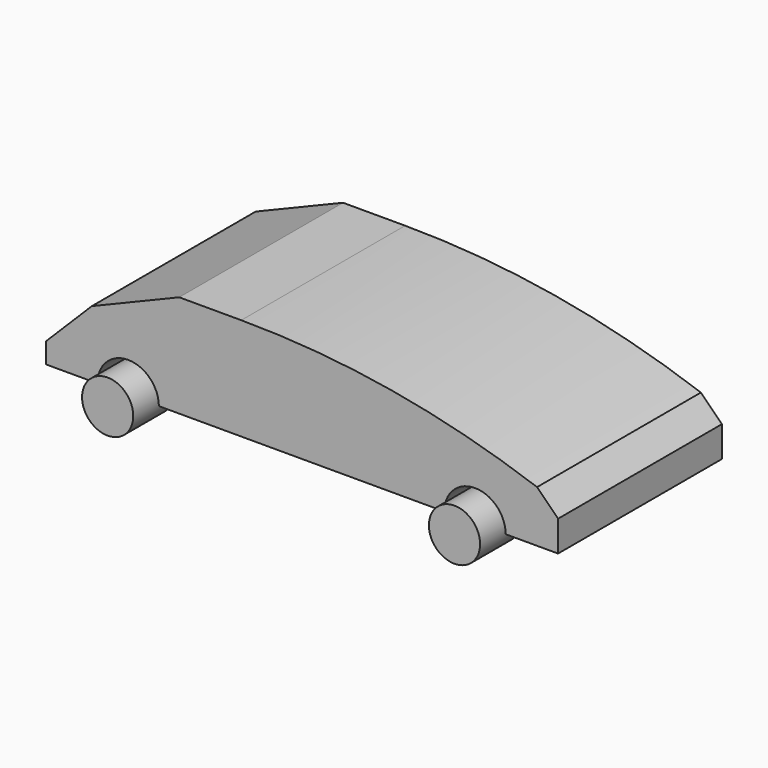
from build123d import *

# Parameters (mm, degrees)
F0_W        = 127
F0_H        = 50.8
F1_DEPTH    = 25.4
F2_SIZE     = 17.78
F3_SIZE     = 17.78
F4_T1_DEPTH = 265.915946003
F5_SIZE     = 20.32
F6_SIZE     = 12.7
F9_DEPTH    = 64.008
F10_DEPTH   = 80.264
F11_DEPTH   = 6.35
F12_R       = 2.54
F13_DEPTH   = 5.08
F15_DEPTH   = 108.712
F16_DEPTH   = 6.35
F17_R       = 2.54
F18_DEPTH   = 5.08
F19_R       = 6.35
F19_R_2     = 2.54
F20_DEPTH   = 6.35
F21_R       = 2.54
F22_DEPTH   = 5.08
F23_DEPTH   = 48.26


# Not quite as in the source:
# - a fillet or chamfer that OpenCascade refuses, or shapes differently, is made with other operations: its cross-section is extruded or revolved along the edge and cut away or added


with BuildPart() as f1:
    # F0 (on Top) → F1 (new body)
    with BuildSketch(Plane.XY):
        with Locations((3.6809762716, -11.9118855059)):
            Rectangle(F0_W, F0_H)
    extrude(amount=F1_DEPTH)

    # F2
    f2_edges = [f1.edges().sort_by_distance(p)[0] for p in [
        (67.180976, -11.911886, 25.4),
    ]]
    chamfer(f2_edges, length=F2_SIZE)

    # F3
    f3_edges = [f1.edges().sort_by_distance(p)[0] for p in [
        (49.400976, -11.911886, 25.4),
    ]]
    chamfer(f3_edges, length=F3_SIZE)

    # F4: fillet of radius 220.4055499979 on 1 edges, made by hand

    # F4_s2 → F4_t1 (cut)
    with BuildSketch(Plane.XZ.offset(-121.0460874956)):
        with BuildLine():
            ThreePointArc((61.9733348411, 12.8276414305), (25.8202104559, 22.2341739644), (-11.402212929, 25.4))
            Line((-11.402212929, 25.4), (31.6209762716, 25.4))
            Line((31.6209762716, 25.4), (61.9733348411, 12.8276414305))
        make_face()
    extrude(amount=F4_T1_DEPTH, mode=Mode.SUBTRACT)

    # F5
    f5_edges = [f1.edges().sort_by_distance(p)[0] for p in [
        (-59.819024, -11.911886, 25.4),
    ]]
    chamfer(f5_edges, length=F5_SIZE)

    # F6
    f6_edges = [f1.edges().sort_by_distance(p)[0] for p in [
        (-39.499024, -11.911886, 25.4),
    ]]
    chamfer(f6_edges, length=F6_SIZE)

    # F8 (on face) → F9 (cut)
    with BuildSketch(Plane(origin=(0, 13.4881144941, 0), x_dir=(-1, 0, 0), z_dir=(0, 1, 0))):
        with BuildLine():
            ThreePointArc((-52.9181478381, 0), (-46.5681478381, 6.35), (-40.2181478381, 0))
            Line((-40.2181478381, 0), (-38.9481478381, 0))
            ThreePointArc((-38.9481478381, 0), (-46.5681478381, 7.62), (-54.1881478381, 0))
            Line((-54.1881478381, 0), (-52.9181478381, 0))
        make_face()
        with BuildLine():
            Line((-52.9181478381, 0), (-40.2181478381, 0))
            ThreePointArc((-40.2181478381, 0), (-46.5681478381, 6.35), (-52.9181478381, 0))
        make_face()
        with BuildLine():
            ThreePointArc((45.8156211138, 0), (39.4656211138, 6.35), (33.1156211138, 0))
            Line((33.1156211138, 0), (45.8156211138, 0))
        make_face()
        with BuildLine():
            ThreePointArc((47.0856211138, 0), (39.4656211138, 7.62), (31.8456211138, 0))
            Line((31.8456211138, 0), (33.1156211138, 0))
            ThreePointArc((33.1156211138, 0), (39.4656211138, 6.35), (45.8156211138, 0))
            Line((45.8156211138, 0), (47.0856211138, 0))
        make_face()
    extrude(amount=-F9_DEPTH, mode=Mode.SUBTRACT)

    # F7 (on face) → F10 (cut)
    with BuildSketch(Plane.XZ.offset(37.3118855059)):
        with BuildLine():
            Line((-45.8156211138, 0), (-33.1156211138, 0))
            ThreePointArc((-33.1156211138, 0), (-39.4656211138, 6.35), (-45.8156211138, 0))
        make_face()
    extrude(amount=-F10_DEPTH, mode=Mode.SUBTRACT)

    # F7 (on face) → F15 (cut)
    with BuildSketch(Plane.XZ.offset(37.3118855059)):
        with BuildLine():
            Line((52.9181478381, 0), (40.2181478381, 0))
            ThreePointArc((40.2181478381, 0), (46.5681478381, -6.35), (52.9181478381, 0))
        make_face()
    extrude(amount=-F15_DEPTH, mode=Mode.SUBTRACT)


with BuildPart() as f11:
    # F7 (on face) → F11 (new body, symmetric)
    with BuildSketch(Plane.XZ.offset(37.3118855059)):
        with BuildLine():
            ThreePointArc((-45.8156211138, 0), (-39.4656211138, -6.35), (-33.1156211138, 0))
            Line((-33.1156211138, 0), (-45.8156211138, 0))
        make_face()
        with BuildLine():
            Line((-45.8156211138, 0), (-33.1156211138, 0))
            ThreePointArc((-33.1156211138, 0), (-39.4656211138, 6.35), (-45.8156211138, 0))
        make_face()
    extrude(amount=F11_DEPTH, both=True)

    # F12 (on face) → F13 (cut)
    with BuildSketch(Plane(origin=(0, -30.9618855059, 0), x_dir=(-1, 0, 0), z_dir=(0, 1, 0))):
        with Locations((39.4656211138, 0)):
            Circle(F12_R)
    extrude(amount=-F13_DEPTH, mode=Mode.SUBTRACT)

    # F23 (add, through all): a face of the model
    f23_faces = [f11.faces().sort_by_distance(p)[0] for p in [
        (-39.4656211138, -36.0418855059, 0),
    ]]


with BuildPart() as f16:
    # F7 (on face) → F16 (new body, symmetric)
    with BuildSketch(Plane.XZ.offset(37.3118855059)):
        with BuildLine():
            Line((52.9181478381, 0), (40.2181478381, 0))
            ThreePointArc((40.2181478381, 0), (46.5681478381, -6.35), (52.9181478381, 0))
        make_face()
        with BuildLine():
            ThreePointArc((52.9181478381, 0), (46.5681478381, 6.35), (40.2181478381, 0))
            Line((40.2181478381, 0), (52.9181478381, 0))
        make_face()
    extrude(amount=F16_DEPTH, both=True)

    # F17 (on face) → F18 (cut)
    with BuildSketch(Plane(origin=(0, -30.9618855059, 0), x_dir=(-1, 0, 0), z_dir=(0, 1, 0))):
        with Locations((-46.5681478381, 0)):
            Circle(F17_R)
    extrude(amount=-F18_DEPTH, mode=Mode.SUBTRACT)

    # F23#2 (add, through all): a face of the model
    f23_2_faces = [f16.faces().sort_by_distance(p)[0] for p in [
        (46.5681478381, -36.0418855059, 0),
    ]]


with BuildPart() as f20:
    # F19 (on face) → F20 (new body, symmetric)
    with BuildSketch(Plane(origin=(0, 13.4881144941, 0), x_dir=(-1, 0, 0), z_dir=(0, 1, 0))):
        with Locations((-46.5681478381, 0)):
            Circle(F19_R)
        with Locations((-46.5681478381, 0)):
            Circle(F19_R_2, mode=Mode.SUBTRACT)
        with Locations((-46.5681478381, 0)):
            Circle(F19_R_2)
    extrude(amount=F20_DEPTH, both=True)


with BuildPart() as f20b:
    # F19 (on face) → F20, piece 2 (new body, symmetric)
    with BuildSketch(Plane(origin=(0, 13.4881144941, 0), x_dir=(-1, 0, 0), z_dir=(0, 1, 0))):
        with Locations((39.4656211138, 0)):
            Circle(F19_R)
        with Locations((39.4656211138, 0)):
            Circle(F19_R_2, mode=Mode.SUBTRACT)
        with Locations((39.4656211138, 0)):
            Circle(F19_R_2)
    extrude(amount=F20_DEPTH, both=True)


with BuildPart() as f22_tool:
    # F21 (on face) → F22 (new body)
    with BuildSketch(Plane.XZ.offset(-7.1381144941)):
        with Locations((-39.4656211138, 0)):
            Circle(F21_R)
        with Locations((46.5681478381, 0)):
            Circle(F21_R)
    extrude(amount=-F22_DEPTH)


with BuildPart() as f20_1:
    add(f20.part)

    # F22: cut by f22_tool
    add(f22_tool.part, mode=Mode.SUBTRACT)


with BuildPart() as f20b_1:
    add(f20b.part)

    # F22: cut by f22_tool
    add(f22_tool.part, mode=Mode.SUBTRACT)


with BuildPart() as f11_1:
    add(f11.part)

    add(f20b_1.part)  # F23 merges F20b
    extrude(f23_faces, amount=F23_DEPTH)


with BuildPart() as f16_1:
    add(f16.part)

    add(f20_1.part)  # F23#2 merges F20
    extrude(f23_2_faces, amount=F23_DEPTH)


solid = Compound([f1.part, f11_1.part, f16_1.part])
